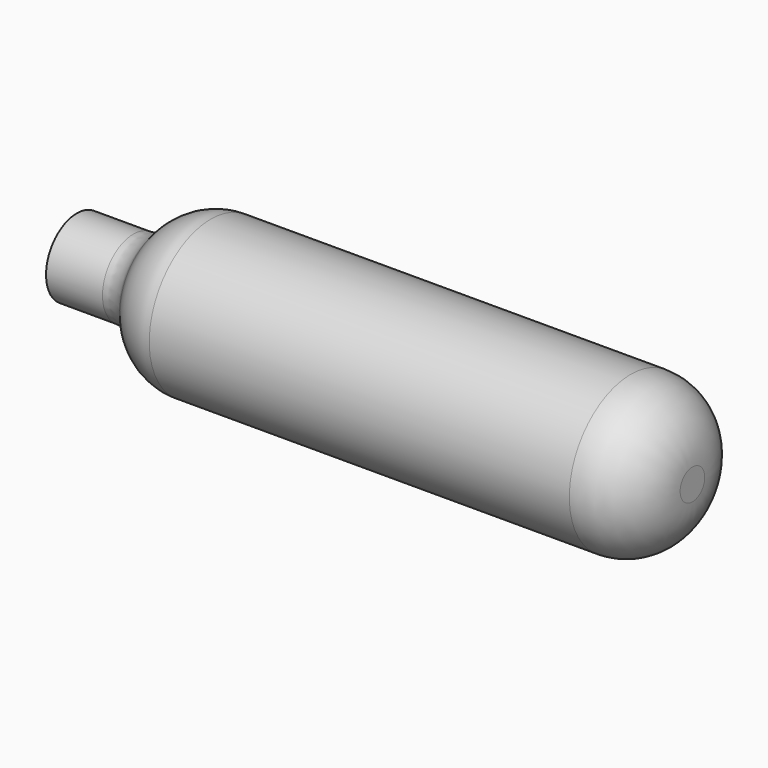
from build123d import *

# Parameters (mm, degrees)
F0_R     = 3.175
F1_DEPTH = 6.35
F2_R     = 6.35
F3_DEPTH = 44.45
F4_R     = 5.08
F6_R     = 2.9585715778


# Not quite as in the source:
# - a fillet or chamfer that OpenCascade refuses, or shapes differently, is made with other operations: its cross-section is extruded or revolved along the edge and cut away or added


with BuildPart() as f1:
    # F0 (on Right) → F1 (new body)
    with BuildSketch(Plane.YZ):
        Circle(F0_R)
    extrude(amount=F1_DEPTH)

    # F2 (on face) → F3 (join)
    with BuildSketch(Plane.YZ.offset(6.35)):
        Circle(F2_R)
    extrude(amount=F3_DEPTH)

    # F4
    f4_edges = [f1.edges().sort_by_distance(p)[0] for p in [
        (50.8, -6.35, 0),
    ]]
    fillet(f4_edges, radius=F4_R)

    # F5: fillet of radius 5.08 on 1 edges, made by hand

    # F5_s1 → F5_t2 (revolve, cut)
    with BuildSketch(Plane.XY):
        with BuildLine():
            ThreePointArc((11.0592860393, 6.35), (8.2194797079, 5.4821134838), (6.35, 3.175))
            Line((6.35, 3.175), (6.35, 6.35))
            Line((6.35, 6.35), (11.0592860393, 6.35))
        make_face()
    revolve(axis=Axis((6.35, 0, 0), (1, 0, 0)), mode=Mode.SUBTRACT)

    # F6
    f6_edges = [f1.edges().sort_by_distance(p)[0] for p in [
        (6.35, -3.175, 0),
    ]]
    fillet(f6_edges, radius=F6_R)


solid = f1.part
